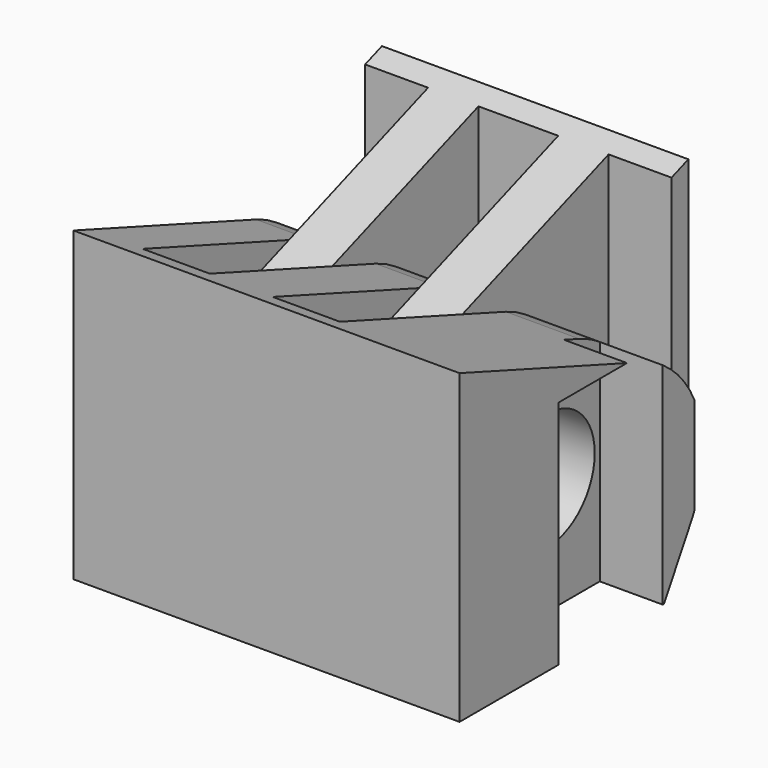
from build123d import *

# Parameters (mm, degrees)
F1_DEPTH      = 25
F2_R          = 2.8
F3_DEPTH      = 7.301
F3_DEPTH_BACK = 11.201
F4_DEPTH      = 7.301
F4_DEPTH_BACK = 11.201
F5_DEPTH      = 7.301
F5_DEPTH_BACK = 11.201
F6_W          = 6.2
F6_H          = 11
F6_R          = 2.8
F7_DEPTH      = 3


with BuildPart() as f1:
    # F0 (on Top) → F1 (new body)
    with BuildSketch(Plane.XY):
        Polygon((7.3, 9.5), (0, 9.5), (-7.3, 9.5), (-7.3, 8.5), (-4.3, 8.5), (-4.3, -6.5), (-1.9, -6.5), (-1.9, 8.5), (0, 8.5), (1.9, 8.5), (1.9, -6.5), (4.3, -6.5), (4.3, 8.5), (7.3, 8.5), align=None)
    extrude(amount=F1_DEPTH)


with BuildPart() as f1b:
    # F0 (on Top) → F1, piece 2 (new body)
    with BuildSketch(Plane.XY):
        Polygon((1.5, 5.5), (0, 5.5), (-1.5, 5.5), (-1.5, -8), (-4.7, -8), (-4.7, 5.5), (-7.2, 5.5), (-7.2, -9), (11.2, -9), (11.2, 5), (7.2, 5), (7.2, 5.5), (4.7, 5.5), (4.7, -8), (1.5, -8), align=None)
    extrude(amount=F1_DEPTH)

    # F2 (on Right) → F3 (cut, two sides)
    with BuildSketch(Plane.YZ) as f3_sk:
        with Locations((0, 5.5)):
            Circle(F2_R)
        with BuildLine():
            ThreePointArc((1.8811107883, 10.6683094143), (4.5053362436, 8.6546703999), (5.5, 5.5))
            ThreePointArc((5.5, 5.5), (5.3125920446, 4.0764952519), (4.7631397208, 2.75))
            Line((4.7631397208, 2.75), (3.1754264805, 0))
            Line((3.1754264805, 0), (37.4948854785, 0))
            Line((37.4948854785, 0), (37.4948854785, 25))
            Line((37.4948854785, 25), (0, 11.3529777486))
            Line((0, 11.3529777486), (1.8811107883, 10.6683094143))
        make_face()
    extrude(amount=-F3_DEPTH, mode=Mode.SUBTRACT)
    extrude(f3_sk.sketch, amount=F3_DEPTH_BACK, mode=Mode.SUBTRACT)


with BuildPart() as f4_tool:
    # F2 (on Right) → F4 (new body, two sides)
    with BuildSketch(Plane.YZ) as f4_sk:
        with Locations((0, 5.5)):
            Circle(F2_R)
        Polygon((-37.4948854785, 25), (0, 11.3529777486), (37.4948854785, 25), align=None)
    extrude(amount=-F4_DEPTH)
    extrude(f4_sk.sketch, amount=F4_DEPTH_BACK)


with BuildPart() as f1_1:
    add(f1.part)

    # F4: cut by f4_tool
    add(f4_tool.part, mode=Mode.SUBTRACT)

    # F2 (on Right) → F5 (cut, two sides)
    with BuildSketch(Plane.YZ) as f5_sk:
        Polygon((-37.4948854785, 25), (0, 11.3529777486), (37.4948854785, 25), align=None)
        with BuildLine():
            ThreePointArc((-4.7631397208, 2.75), (-5.1683094143, 7.3811107883), (-1.8811107883, 10.6683094143))
            Line((-1.8811107883, 10.6683094143), (0, 11.3529777486))
            Line((0, 11.3529777486), (-37.4948854785, 25))
            Line((-37.4948854785, 25), (-37.4948854785, 0))
            Line((-37.4948854785, 0), (-3.1754264805, 0))
            Line((-3.1754264805, 0), (-4.7631397208, 2.75))
        make_face()
    extrude(amount=-F5_DEPTH, mode=Mode.SUBTRACT)
    extrude(f5_sk.sketch, amount=F5_DEPTH_BACK, mode=Mode.SUBTRACT)


with BuildPart() as f1b_1:
    add(f1b.part)

    # F4: cut by f4_tool
    add(f4_tool.part, mode=Mode.SUBTRACT)

    # F6 (on face) → F7 (cut)
    with BuildSketch(Plane.YZ.offset(11.2)):
        with Locations((0, 5.5)):
            Rectangle(F6_W, F6_H)
        with Locations((0, 5.5)):
            Circle(F6_R, mode=Mode.SUBTRACT)
    extrude(amount=-F7_DEPTH, mode=Mode.SUBTRACT)


solid = Compound([f1_1.part, f1b_1.part])
